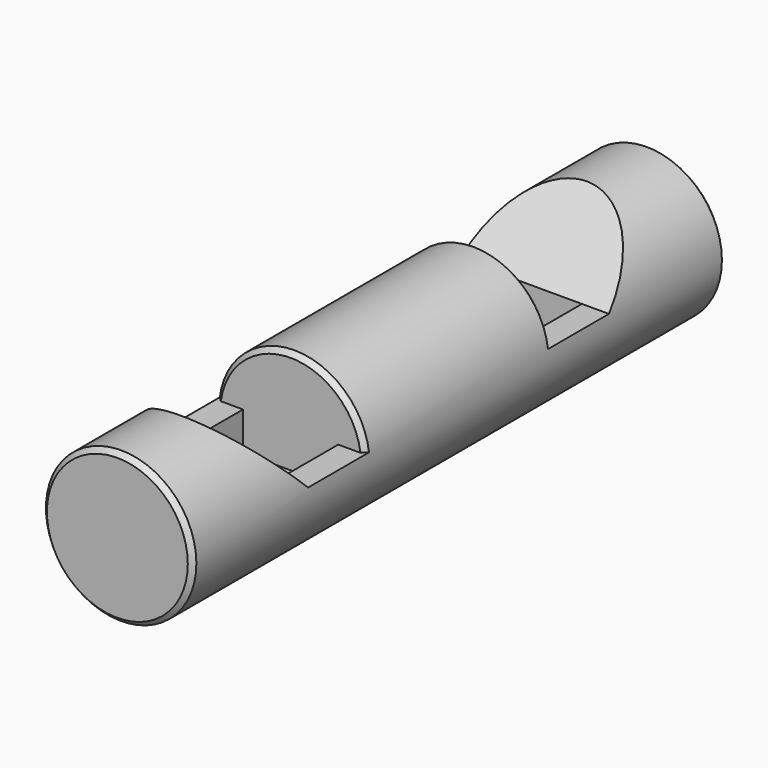
from build123d import *

# Parameters (mm, degrees)
F0_R     = 158
F1_DEPTH = 1400
F3_DEPTH = 158.001
F4_DEPTH = 158.001
F5_SIZE  = 137.99999
F6_SIZE  = 137.99999
F9_DEPTH = 80
F10_SIZE = 10
F11_SIZE = 10


# Not quite as in the source:
# - a fillet or chamfer is up to 0.001 mm smaller than in the source, because OpenCascade refuses the exact size


with BuildPart() as f1:
    # F0 (on Front) → F1 (new body)
    with BuildSketch(Plane.XZ):
        Circle(F0_R)
    extrude(amount=-F1_DEPTH)

    # F2 (on Right) → F3 (cut, through all)
    with BuildSketch(Plane.YZ):
        Polygon((167, 20), (390, 20), (455, 20), (455, 158), (167, 158), align=None)
        Polygon((945, 158), (945, 20), (1010, 20), (1233, 20), (1233, 158), align=None)
    extrude(amount=-F3_DEPTH, mode=Mode.SUBTRACT)

    # F4 (cut, through all): faces of the model
    f4_faces = [f1.faces().sort_by_distance(p)[0] for p in [
        (0, 1089, 89),
        (0, 311, 89),
    ]]
    extrude(f4_faces, amount=-F4_DEPTH, mode=Mode.SUBTRACT)

    # F5 (size 138 in the source; OpenCascade refuses exactly that, so slightly less here)
    f5_edges = [f1.edges().sort_by_distance(p)[0] for p in [
        (0, 1233, 20),
    ]]
    chamfer(f5_edges, length=F5_SIZE)

    # F6 (size 138 in the source; OpenCascade refuses exactly that, so slightly less here)
    f6_edges = [f1.edges().sort_by_distance(p)[0] for p in [
        (0, 167, 20),
    ]]
    chamfer(f6_edges, length=F6_SIZE)

    # F7 (on face) + F8 (on face) → F9 (cut)
    with BuildSketch(Plane.XY.offset(20)):
        Polygon((100, 1095), (0, 1095), (-100, 1095), (-100, 945), (100, 945), align=None)
    with BuildSketch(Plane.XY.offset(20)):
        Polygon((-100, 305), (0, 305), (100, 305), (100, 455), (-100, 455), align=None)
    extrude(amount=-F9_DEPTH, mode=Mode.SUBTRACT)

    # F10
    f10_edges = [f1.edges().sort_by_distance(p)[0] for p in [
        (-158, 0, 0),
        (-158, 1400, 0),
    ]]
    chamfer(f10_edges, length=F10_SIZE)

    # F11
    f11_edges = [f1.edges().sort_by_distance(p)[0] for p in [
        (0, 455, 158),
        (0, 945, 158),
    ]]
    chamfer(f11_edges, length=F11_SIZE)


solid = f1.part
